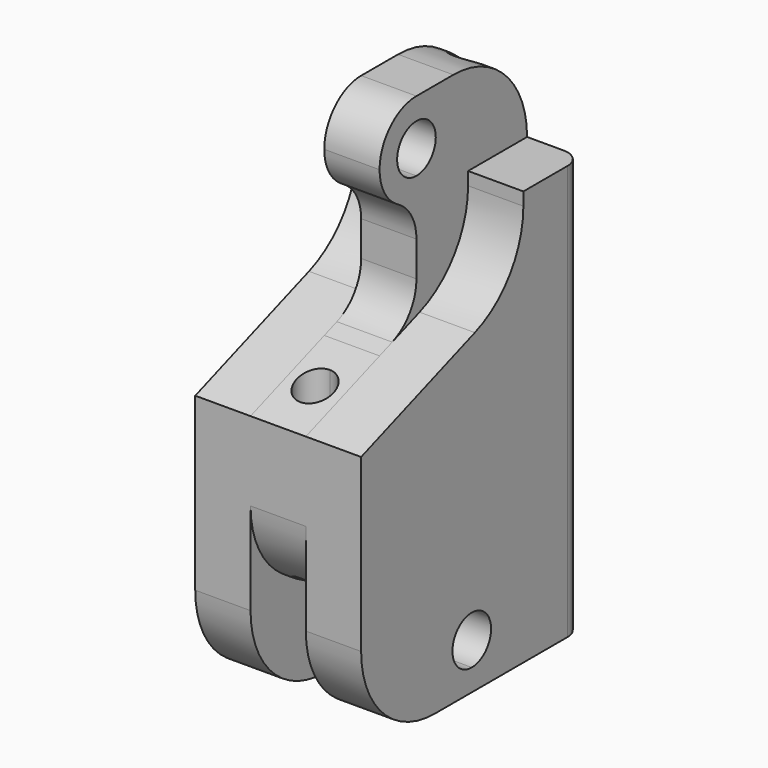
from build123d import *

# Parameters (mm, degrees)
F1_DEPTH     = 15
F3_DEPTH     = 6
F5_DEPTH     = 18
F6_R         = 10
F9_DEPTH     = 6
F10_DEPTH    = 6
F11_R        = 2
F13_DEPTH    = 6
F15_R        = 10
F19_DEPTH    = 50.001
F21_DEPTH    = 45.001
F23_DEPTH    = 6
F24_T1_DEPTH = 6


# Not quite as in the source:
# - a fillet or chamfer that OpenCascade refuses, or shapes differently, is made with other operations: its cross-section is extruded or revolved along the edge and cut away or added


with BuildPart() as f1:
    # F0 (on Front) → F1 (new body, symmetric)
    with BuildSketch(Plane.XZ):
        Polygon((9, -17.5), (9, 17.5), (3, 17.5), (3, 27.5), (-3, 27.5), (-3, 17.5), (-9, 17.5), (-9, -17.5), (-9, -27.5), (-3, -27.5), (-3, -17.5), (3, -17.5), (3, -27.5), (9, -27.5), align=None)
    extrude(amount=F1_DEPTH, both=True)

    # F2 (on face) → F3 (cut)
    with BuildSketch(Plane(origin=(-3, 0, 0), x_dir=(0, -1, 0), z_dir=(-1, 0, 0))):
        with BuildLine():
            ThreePointArc((0, 25.12), (-2.62, 22.5), (0, 19.88))
            Line((0, 19.88), (0, 25.12))
        make_face()
        with BuildLine():
            Line((0, 25.12), (0, 19.88))
            ThreePointArc((0, 19.88), (1.8526197667, 20.6473802333), (2.62, 22.5))
            ThreePointArc((2.62, 22.5), (1.8526197667, 24.3526197667), (0, 25.12))
        make_face()
    extrude(amount=-F3_DEPTH, mode=Mode.SUBTRACT)

    # F4 (on face) → F5 (cut)
    with BuildSketch(Plane(origin=(-9, 0, 0), x_dir=(0, -1, 0), z_dir=(-1, 0, 0))):
        with BuildLine():
            ThreePointArc((0, -25.12), (1.8526197667, -24.3526197667), (2.62, -22.5))
            ThreePointArc((2.62, -22.5), (-1.8526197667, -20.6473802333), (0, -25.12))
        make_face()
    extrude(amount=-F5_DEPTH, mode=Mode.SUBTRACT)

    # F6
    f6_edges = [f1.edges().sort_by_distance(p)[0] for p in [
        (0, 15, 27.5),
        (0, -15, 27.5),
        (6, -15, -27.5),
        (-6, -15, -27.5),
    ]]
    fillet(f6_edges, radius=F6_R)

    # F8 (on face) → F9 (cut)
    with BuildSketch(Plane(origin=(-9, 0, 0), x_dir=(0, -1, 0), z_dir=(-1, 0, 0))):
        with BuildLine():
            ThreePointArc((-7, 16.0872004348), (-5.1915204429, 10.3514360713), (-0.4202014333, 6.690274227))
            Line((-0.4202014333, 6.690274227), (15, 1.0777798989))
            Line((15, 1.0777798989), (15, 17.5))
            Line((15, 17.5), (-7, 17.5))
            Line((-7, 17.5), (-7, 16.0872004348))
        make_face()
    extrude(amount=-F9_DEPTH, mode=Mode.SUBTRACT)

    # F7 (on face) → F10 (cut)
    with BuildSketch(Plane.YZ.offset(9)):
        with BuildLine():
            Line((7, 17.5), (-15, 17.5))
            Line((-15, 17.5), (-15, 1.07778))
            Line((-15, 1.07778), (0.4202014333, 6.6902743281))
            ThreePointArc((0.4202014333, 6.6902743281), (5.1915204429, 10.3514361724), (7, 16.087200536))
            Line((7, 16.087200536), (7, 17.5))
        make_face()
    extrude(amount=-F10_DEPTH, mode=Mode.SUBTRACT)

    # F11
    f11_edges = [f1.edges().sort_by_distance(p)[0] for p in [
        (9, 15, -5),
        (-9, 15, -5),
    ]]
    fillet(f11_edges, radius=F11_R)

    # F12 (on face) → F13 (cut)
    with BuildSketch(Plane(origin=(-3, 0, 0), x_dir=(0, -1, 0), z_dir=(-1, 0, 0))):
        with BuildLine():
            Line((5, 27.5), (0, 27.5))
            ThreePointArc((0, 27.5), (3.5355339059, 26.0355339059), (5, 22.5))
            Line((5, 22.5), (5, 4.7174822415))
            Line((5, 4.7174822415), (15, 1.0777798989))
            Line((15, 1.0777798989), (15, 17.5))
            ThreePointArc((15, 17.5), (12.0710678119, 24.5710678119), (5, 27.5))
        make_face()
    extrude(amount=-F13_DEPTH, mode=Mode.SUBTRACT)

    # F15
    f15_edges = [f1.edges().sort_by_distance(p)[0] for p in [
        (0, -15, -17.5),
    ]]
    fillet(f15_edges, radius=F15_R)

    # F18 (on face) → F19 (cut, through all)
    with BuildSketch(Plane.XY.offset(22.5)):
        with BuildLine():
            ThreePointArc((2, -10), (1.4142135624, -8.5857864376), (0, -8))
            Line((0, -8), (0, -12))
            ThreePointArc((0, -12), (1.4142135624, -11.4142135624), (2, -10))
        make_face()
        with BuildLine():
            Line((0, -12), (0, -8))
            ThreePointArc((0, -8), (-2, -10), (0, -12))
        make_face()
    extrude(amount=-F19_DEPTH, mode=Mode.SUBTRACT)

    # F20 (on face) → F21 (cut, through all)
    with BuildSketch(Plane(origin=(0, 0, -17.5), x_dir=(1, 0, 0), z_dir=(0, 0, -1))):
        with BuildLine():
            ThreePointArc((0, -9), (-2, -11), (0, -13))
            Line((0, -13), (0, -11))
            Line((0, -11), (0, -9))
        make_face()
        with BuildLine():
            Line((0, -11), (0, -13))
            ThreePointArc((0, -13), (1.4142135624, -12.4142135624), (2, -11))
            ThreePointArc((2, -11), (1.4142135624, -9.5857864376), (0, -9))
            Line((0, -9), (0, -11))
        make_face()
    extrude(amount=-F21_DEPTH, mode=Mode.SUBTRACT)

    # F22 (on face) → F23 (cut)
    with BuildSketch(Plane.YZ.offset(3)):
        with BuildLine():
            ThreePointArc((0, 17.5), (-3.5355339059, 18.9644660941), (-5, 22.5))
            Line((-5, 22.5), (-5, 4.7174822415))
            Line((-5.0000000325, 4.7174823308), (0, 6.537333514))
            Line((0, 6.537333514), (0, 17.5))
        make_face()
    extrude(amount=-F23_DEPTH, mode=Mode.SUBTRACT)

    # F24: fillet of radius 5 on 2 edges, made by hand

    # F24_s2 → F24_t1 (join)
    with BuildSketch(Plane.YZ.offset(-3)):
        with BuildLine():
            ThreePointArc((-2.5, 18.1698729811), (-0.6698729811, 16.3397459622), (0, 13.8397459622))
            Line((0, 13.8397459622), (0, 17.5))
            ThreePointArc((0, 17.5), (-1.2940952255, 17.6703708686), (-2.5, 18.1698729811))
        make_face()
        with BuildLine():
            ThreePointArc((-3.2898992834, 5.3399081011), (-0.9042397786, 7.1704890233), (0, 10.038371205))
            Line((0, 10.038371205), (0, 6.537333514))
            Line((0, 6.537333514), (-3.2898992834, 5.3399081011))
        make_face()
    extrude(amount=F24_T1_DEPTH)


solid = f1.part
